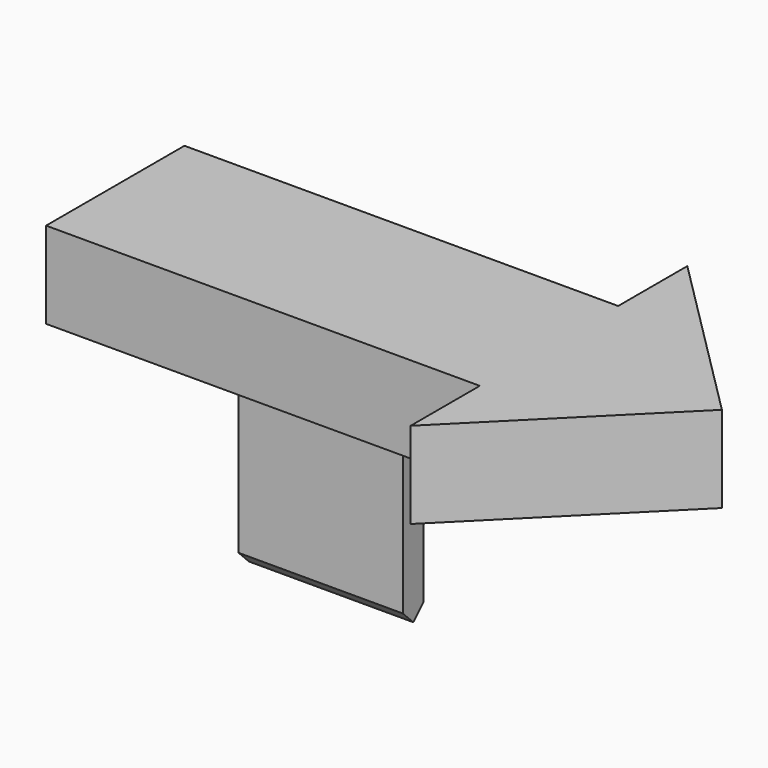
from build123d import *

# Parameters (mm, degrees)
F1_DEPTH    = 5
F2_W        = 9.5
F2_H        = 1.5
F3_DEPTH    = 12
F4_T1_DEPTH = 14.6433659759


# Not quite as in the source:
# - a fillet or chamfer that OpenCascade refuses, or shapes differently, is made with other operations: its cross-section is extruded or revolved along the edge and cut away or added


with BuildPart() as f1:
    # F0 (on Top) → F1 (new body)
    with BuildSketch(Plane.XY):
        Polygon((-2.5628354418, 5), (-27.6419919184, 5), (-27.6419919184, -5), (-2.5628354418, -5), (-2.5628354418, -10), (7.4371645582, 0), (-2.5628354418, 10), align=None)
    extrude(amount=F1_DEPTH)

    # F2 (on face) → F3 (join)
    with BuildSketch(Plane(origin=(0, 0, 0), x_dir=(1, 0, 0), z_dir=(0, 0, -1))):
        with Locations((-15.3186318129, -0.1973686223)):
            Rectangle(F2_W, F2_H)
    extrude(amount=F3_DEPTH)

    # F4: chamfer of 1 on 2 edges, made by hand

    # F4_s2 → F4_t1 (cut)
    with BuildSketch(Plane.YZ.offset(-22.6403148009)):
        Polygon((0.9473686223, -11), (-0.0526313777, -12), (0.9473686223, -12), align=None)
        Polygon((-0.5526313777, -11), (0.4473686223, -12), (-0.5526313777, -12), align=None)
    extrude(amount=F4_T1_DEPTH, mode=Mode.SUBTRACT)


solid = f1.part
